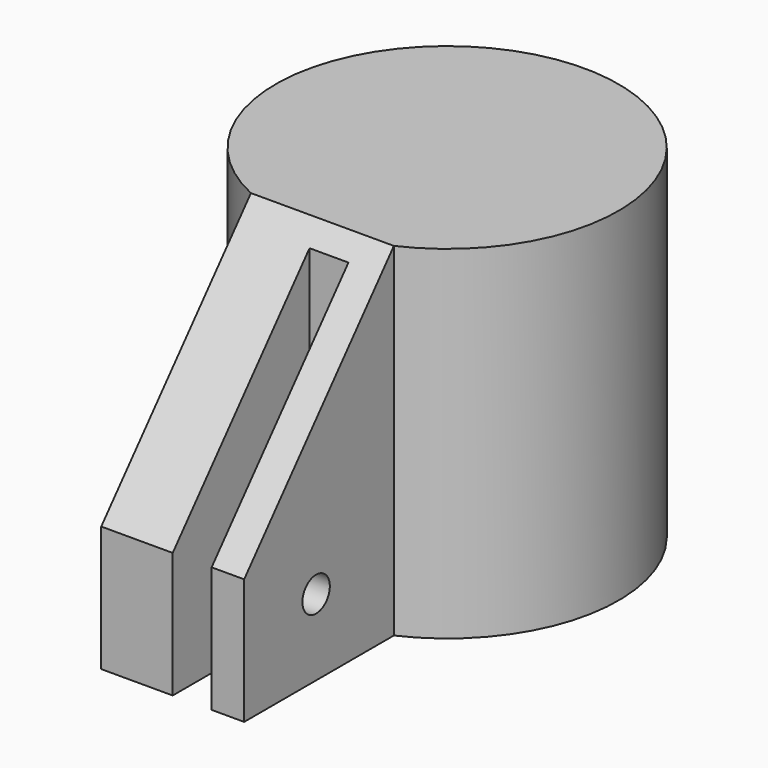
from build123d import *

# Parameters (mm, degrees)
F0_R      = 30
F1_DEPTH  = 60
F2_W      = 25
F2_H      = 60
F3_DEPTH  = 60
F5_DEPTH  = 25
F6_W      = 6.8101426587
F6_H      = 36.6509445012
F5_FACE_W = 25
F5_FACE_H = 50.1833343375
F7_DEPTH  = 114.6
F9_D      = 6


# Not quite as in the source:
# - a feature of the source that left no trace in its solid (it failed there, or was rolled back) is left out
# - a feature names something its author has since deleted; it is built from what else it names


with BuildPart() as f1:
    # F0 (on Top) → F1 (new body)
    with BuildSketch(Plane.XY):
        Circle(F0_R)
    extrude(amount=F1_DEPTH)

    # F2 (on Front) → F3 (join)
    with BuildSketch(Plane.XZ):
        with Locations((0, 30)):
            Rectangle(F2_W, F2_H)
    extrude(amount=F3_DEPTH)

    # F4 (on face) → F5 (cut)
    with BuildSketch(Plane.YZ.offset(12.5)):
        Polygon((-60, 21.9575148076), (-27.2717802866, 60), (-60, 60), align=None)
    extrude(amount=-F5_DEPTH, mode=Mode.SUBTRACT)

    # F6 (on Top) + F5_face (on face) → F7 (cut)
    with BuildSketch(Plane.XY):
        with Locations((3.4050713293, -48.4139155596)):
            Rectangle(F6_W, F6_H)
    with BuildSketch(Plane(origin=(0, -43.6358901433, 40.9787574038), x_dir=(1, 0, 0), z_dir=(0, -0.7580700983, 0.6521730799))):
        Rectangle(F5_FACE_W, F5_FACE_H)
    extrude(amount=F7_DEPTH, dir=(0, 0, 1), mode=Mode.SUBTRACT)

    # F9 (through all)
    with Locations(Plane.YZ.offset(12.5)):
        with Locations((-44.2717802866, 13.2831530645)):
            Hole(F9_D / 2)


solid = f1.part
